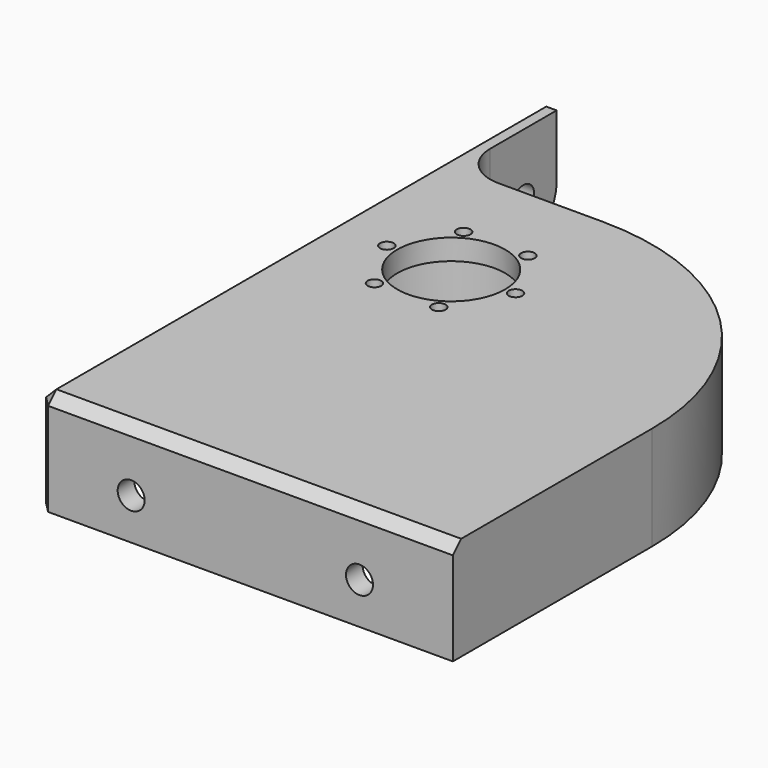
from build123d import *

# Parameters (mm, degrees)
F0_R     = 21.25
F0_R_2   = 1.65
F0_R_3   = 13
F1_DEPTH = 5
F2_DEPTH = 20
F3_W     = 5
F3_H     = 25
F4_DEPTH = 30
F6_R     = 3.25
F7_DEPTH = 25
F5_R     = 3
F5_R_2   = 3.25
F8_DEPTH = 25
F9_SIZE  = 2.5
F10_R    = 10


# Not quite as in the source:
# - a feature names something its author has since deleted; it is built from what else it names


with BuildPart() as f1:
    # F0 (on Top) → F1 (new body)
    with BuildSketch(Plane.XY):
        with BuildLine():
            Line((30, 60), (5, 60))
            Line((5, 60), (5, 5))
            Line((5, 5), (95, 5))
            Line((95, 5), (95, 59.7859807312))
            ThreePointArc((95, 59.7859807312), (84.7139923095, 92.0261844448), (57.5, 112.1416340365))
            Line((57.5, 112.1416340365), (57.5, 87.5))
            ThreePointArc((57.5, 87.5), (49.4454364826, 68.0545635174), (30, 60))
        make_face()
        with BuildLine():
            Line((40, 120), (5, 120))
            Line((5, 120), (5, 60))
            Line((5, 60), (30, 60))
            ThreePointArc((30, 60), (49.4454364826, 68.0545635174), (57.5, 87.5))
            Line((57.5, 87.5), (57.5, 112.1416340365))
            ThreePointArc((57.5, 112.1416340365), (84.7139923095, 92.0261844448), (95, 59.7859807312))
            Line((95, 59.7859807312), (95, 5))
            Line((95, 5), (100, 5))
            Line((100, 5), (100, 60))
            ThreePointArc((100, 60), (82.4264068712, 102.4264068712), (40, 120))
        make_face()
        with Locations((30, 87)):
            Circle(F0_R, mode=Mode.SUBTRACT)
        with Locations((30, 87)):
            Circle(F0_R)
        with Locations((22.25, 73.5766062413)):
            Circle(F0_R_2, mode=Mode.SUBTRACT)
        with Locations((14.5, 87)):
            Circle(F0_R_2, mode=Mode.SUBTRACT)
        with Locations((37.75, 73.5766062413)):
            Circle(F0_R_2, mode=Mode.SUBTRACT)
        with Locations((30, 87)):
            Circle(F0_R_3, mode=Mode.SUBTRACT)
        with Locations((45.5, 87)):
            Circle(F0_R_2, mode=Mode.SUBTRACT)
        with Locations((22.25, 100.4233937587)):
            Circle(F0_R_2, mode=Mode.SUBTRACT)
        with Locations((37.75, 100.4233937587)):
            Circle(F0_R_2, mode=Mode.SUBTRACT)
        Polygon((0, 120), (0, 0), (100, 0), (100, 5), (95, 5), (5, 5), (5, 60), (5, 120), align=None)
    extrude(amount=F1_DEPTH)

    # F0 (on Top) → F2 (join)
    with BuildSketch(Plane.XY):
        Polygon((0, 120), (0, 0), (100, 0), (100, 5), (95, 5), (5, 5), (5, 60), (5, 120), align=None)
        with BuildLine():
            Line((40, 120), (5, 120))
            Line((5, 120), (5, 60))
            Line((5, 60), (30, 60))
            ThreePointArc((30, 60), (49.4454364826, 68.0545635174), (57.5, 87.5))
            Line((57.5, 87.5), (57.5, 112.1416340365))
            ThreePointArc((57.5, 112.1416340365), (84.7139923095, 92.0261844448), (95, 59.7859807312))
            Line((95, 59.7859807312), (95, 5))
            Line((95, 5), (100, 5))
            Line((100, 5), (100, 60))
            ThreePointArc((100, 60), (82.4264068712, 102.4264068712), (40, 120))
        make_face()
        with Locations((30, 87)):
            Circle(F0_R, mode=Mode.SUBTRACT)
    extrude(amount=-F2_DEPTH)

    # F3 (on face) → F4 (join)
    with BuildSketch(Plane(origin=(0, 120, 0), x_dir=(-1, 0, 0), z_dir=(0, 1, 0))):
        with Locations((-2.5, -7.5)):
            Rectangle(F3_W, F3_H)
    extrude(amount=F4_DEPTH)

    # F6 (on face) → F7 (cut)
    with BuildSketch(Plane.XZ):
        with Locations((22.5, -10)):
            Circle(F6_R)
        with Locations((77.5, -10)):
            Circle(F6_R)
    extrude(amount=-F7_DEPTH, mode=Mode.SUBTRACT)

    # F5 (on face) → F8 (cut)
    with BuildSketch(Plane(origin=(0, 0, 0), x_dir=(0, -1, 0), z_dir=(-1, 0, 0))):
        with Locations((-22.5, -10)):
            Circle(F5_R)
        with Locations((-140, -10)):
            Circle(F5_R_2)
    extrude(amount=-F8_DEPTH, mode=Mode.SUBTRACT)

    # F9
    f9_edges = [f1.edges().sort_by_distance(p)[0] for p in [
        (50, 0, 5),
        (0, 75, 5),
        (0, 0, -7.5),
    ]]
    chamfer(f9_edges, length=F9_SIZE)

    # F10
    f10_edges = [f1.edges().sort_by_distance(p)[0] for p in [
        (5, 5, -10),
        (5, 60, -10),
        (57.5, 112.141634, -10),
        (95, 5, -10),
        (5, 120, -7.5),
        (2.5, 150, -20),
    ]]
    fillet(f10_edges, radius=F10_R)


solid = f1.part
